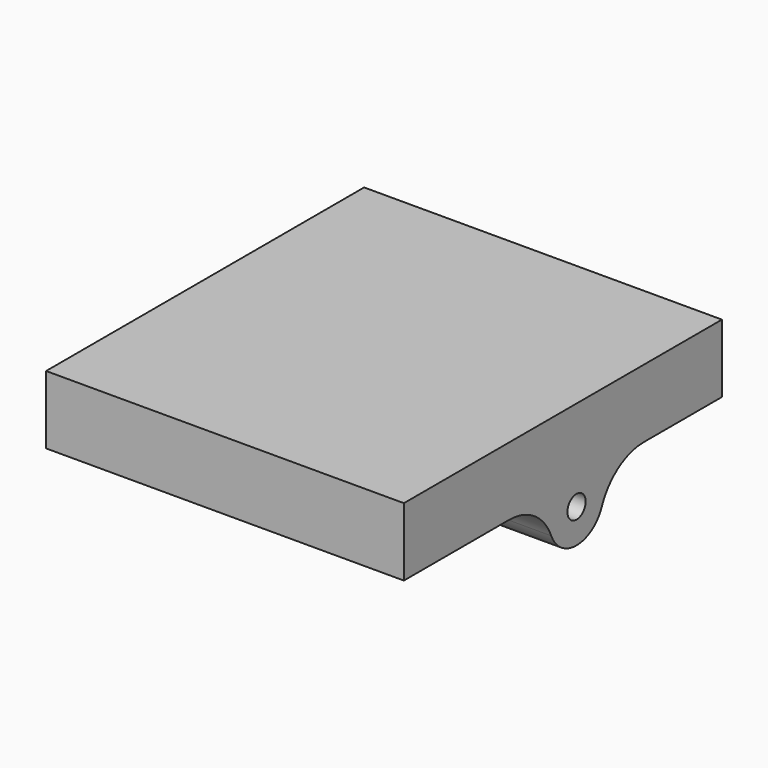
from build123d import *

# Parameters (mm, degrees)
F0_W     = 31.5
F0_H     = 35
F1_DEPTH = 6
F3_DEPTH = 31.5
F4_R     = 5


# Not quite as in the source:
# - a feature of the source that left no trace in its solid (it failed there, or was rolled back) is left out


with BuildPart() as f1:
    # F0 (on Top) → F1 (new body)
    with BuildSketch(Plane.XY):
        with Locations((15.75, 17.5)):
            Rectangle(F0_W, F0_H)
    extrude(amount=F1_DEPTH)

    # F2 (on face) → F3 (join, through all)
    with BuildSketch(Plane.YZ.offset(31.5)):
        with BuildLine():
            Line((22, -2), (22, 0))
            Line((22, 0), (16, 0))
            Line((16, 0), (16, -2))
            Line((16, -2), (18, -2))
            ThreePointArc((18, -2), (19, -1), (20, -2))
            Line((20, -2), (22, -2))
        make_face()
        with BuildLine():
            ThreePointArc((16, -2), (19, -5), (22, -2))
            Line((22, -2), (20, -2))
            ThreePointArc((20, -2), (19, -3), (18, -2))
            Line((18, -2), (16, -2))
        make_face()
    extrude(amount=-F3_DEPTH)

    # F4
    f4_edges = [f1.edges().sort_by_distance(p)[0] for p in [
        (15.75, 22, 0),
        (15.75, 16, 0),
    ]]
    fillet(f4_edges, radius=F4_R)


solid = f1.part
